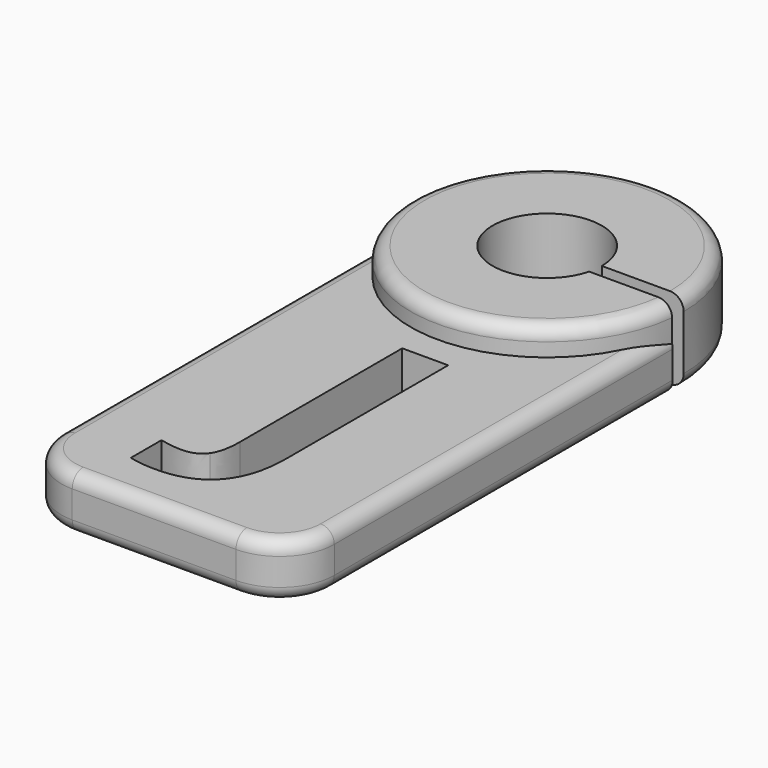
from build123d import *

# Parameters (mm, degrees)
F1_DEPTH     = 3
F2_DEPTH     = 2
F3_R         = 2
F4_T1_DEPTH  = 16.75
F4_T3_DEPTH  = 6
F4_T5_DEPTH  = 16
F4_T10_DEPTH = 16.75
F4_S11_R     = 5
F4_T12_DEPTH = 10
F4_T14_ANGLE = 359.64
F4_T18_DEPTH = 19.75
F4_S19_R     = 5
F4_T20_DEPTH = 11
F4_T22_ANGLE = 90
F4_T24_ANGLE = 90
F4_T26_ANGLE = 90
F4_T28_ANGLE = 180
F4_T30_ANGLE = 90


# Not quite as in the source:
# - a fillet or chamfer that OpenCascade refuses, or shapes differently, is made with other operations: its cross-section is extruded or revolved along the edge and cut away or added


with BuildPart() as f1:
    # F0 (on Top) → F1 (new body)
    with BuildSketch(Plane.XY):
        with BuildLine():
            Line((2, 0), (5, 0))
            ThreePointArc((5, 0), (0, 5), (-5, 0))
            ThreePointArc((-5, 0), (-0.2503138753, -4.9937303656), (4.9749371855, -0.5))
            Line((4.9749371855, -0.5), (1.9364916731, -0.5))
            ThreePointArc((1.9364916731, -0.5), (-1.9840593925, 0.252008585), (2, 0))
        make_face()
    extrude(amount=F1_DEPTH)

    # F0 (on Top) → F2 (join)
    with BuildSketch(Plane.XY):
        with BuildLine():
            ThreePointArc((4.9749371855, -0.5), (-0.2503138753, -4.9937303656), (-5, 0))
            Line((-5, 0), (-5, -18))
            Line((-5, -18), (5, -18))
            Line((5, -18), (5, -0.5))
            Line((5, -0.5), (4.9749371855, -0.5))
        make_face()
        with BuildLine():
            add(Edge.make_bspline(
                [(0.578588878, -15.5900442691), (-0.0559597331, -16.3174748247), (-1.2990152887, -16.3174748247)],
                knots=[0, 0, 0, 1, 1, 1], degree=2))
            add(Edge.make_bspline(
                [(-1.2990152887, -16.3174748247), (-1.8684597331, -16.3174748247), (-2.2920708442, -16.197683158)],
                knots=[0, 0, 0, 1, 1, 1], degree=2))
            Line((-2.2920708442, -16.197683158), (-2.2920708442, -14.7983776025))
            add(Edge.make_bspline(
                [(-2.2920708442, -14.7983776025), (-1.8580430665, -14.9060164914), (-1.5004041776, -14.9060164914)],
                knots=[0, 0, 0, 1, 1, 1], degree=2))
            add(Edge.make_bspline(
                [(-1.5004041776, -14.9060164914), (-0.9465847331, -14.9060164914), (-0.7078694553, -14.5613984358)],
                knots=[0, 0, 0, 1, 1, 1], degree=2))
            add(Edge.make_bspline(
                [(-0.7078694553, -14.5613984358), (-0.4691541776, -14.2167803802), (-0.4691541776, -13.4841414914)],
                knots=[0, 0, 0, 1, 1, 1], degree=2))
            Line((-0.4691541776, -13.4841414914), (-0.4691541776, -6.0518498247))
            Line((-0.4691541776, -6.0518498247), (1.2131374891, -6.0518498247))
            Line((1.2131374891, -6.0518498247), (1.2131374891, -13.4737248247))
            add(Edge.make_bspline(
                [(1.2131374891, -13.4737248247), (1.2131374891, -14.8626137136), (0.578588878, -15.5900442691)],
                knots=[0, 0, 0, 1, 1, 1], degree=2))
        make_face(mode=Mode.SUBTRACT)
    extrude(amount=F2_DEPTH)

    # F3
    f3_edges = [f1.edges().sort_by_distance(p)[0] for p in [
        (-5, -18, 1),
        (5, -18, 1),
    ]]
    fillet(f3_edges, radius=F3_R)

    # F4: fillet of radius 0.5 on 12 edges, made by hand

    # F4_s2 → F4_t1 (cut)
    with BuildSketch(Plane.XZ.offset(-0.75)):
        with BuildLine():
            ThreePointArc((5, 0.5), (4.8535533906, 0.1464466094), (4.5, 0))
            Line((4.5, 0), (5, 0))
            Line((5, 0), (5, 0.5))
        make_face()
    extrude(amount=F4_T1_DEPTH, mode=Mode.SUBTRACT)

    # F4_s4 → F4_t3 (cut)
    with BuildSketch(Plane.YZ.offset(-3)):
        with BuildLine():
            ThreePointArc((-17.5, 2), (-17.8535533906, 1.8535533906), (-18, 1.5))
            Line((-18, 1.5), (-18, 2))
            Line((-18, 2), (-17.5, 2))
        make_face()
        with BuildLine():
            ThreePointArc((-18, 0.5), (-17.8535533906, 0.1464466094), (-17.5, 0))
            Line((-17.5, 0), (-18, 0))
            Line((-18, 0), (-18, 0.5))
        make_face()
    extrude(amount=F4_T3_DEPTH, mode=Mode.SUBTRACT)

    # F4_s6 → F4_t5 (cut)
    with BuildSketch(Plane.XZ):
        with BuildLine():
            ThreePointArc((-5, 0.5), (-4.8535533906, 0.1464466094), (-4.5, 0))
            Line((-4.5, 0), (-5, 0))
            Line((-5, 0), (-5, 0.5))
        make_face()
    extrude(amount=F4_T5_DEPTH, mode=Mode.SUBTRACT)


with BuildPart() as f4_tool8:
    # F4_s9 → F4_t10 (new body)
    with BuildSketch(Plane.XZ.offset(16)):
        with BuildLine():
            ThreePointArc((4.5, 2), (4.8535533906, 1.8535533906), (5, 1.5))
            Line((5, 1.5), (5, 2))
            Line((5, 2), (4.5, 2))
        make_face()
    extrude(amount=-F4_T10_DEPTH)

    # F4_s11 → F4_t12 (cut, symmetric)
    with BuildSketch(Plane.XY.offset(1.8)):
        Circle(F4_S11_R)
    extrude(amount=F4_T12_DEPTH, both=True, mode=Mode.SUBTRACT)


with BuildPart() as f1_1:
    add(f1.part)

    # F4_t7: cut F4_tool8
    add(f4_tool8.part, mode=Mode.SUBTRACT)

    # F4_s13 → F4_t14 (revolve, cut)
    with BuildSketch(Plane(origin=(0, 0, 0), x_dir=(0, 0, 1), z_dir=(0.0532001762, 0.9985838679, 0))):
        with BuildLine():
            ThreePointArc((2.5, 5), (2.8535533906, 4.8535533906), (3, 4.5))
            Line((3, 4.5), (3, 5))
            Line((3, 5), (2.5, 5))
        make_face()
    revolve(axis=Axis((0, 0, 3), (0, 0, -1)), revolution_arc=F4_T14_ANGLE, mode=Mode.SUBTRACT)


with BuildPart() as f4_tool16:
    # F4_s17 → F4_t18 (new body)
    with BuildSketch(Plane.XZ.offset(-3.75)):
        with BuildLine():
            ThreePointArc((-4.5, 2), (-4.8535533906, 1.8535533906), (-5, 1.5))
            Line((-5, 1.5), (-5, 2))
            Line((-5, 2), (-4.5, 2))
        make_face()
    extrude(amount=F4_T18_DEPTH)

    # F4_s19 → F4_t20 (cut, symmetric)
    with BuildSketch(Plane.XY.offset(1.8)):
        Circle(F4_S19_R)
    extrude(amount=F4_T20_DEPTH, both=True, mode=Mode.SUBTRACT)


with BuildPart() as f1_2:
    add(f1_1.part)

    # F4_t15: cut F4_tool16
    add(f4_tool16.part, mode=Mode.SUBTRACT)

    # F4_s21 → F4_t22 (revolve, cut)
    with BuildSketch(Plane.YZ.offset(-3)):
        with BuildLine():
            ThreePointArc((-17.5, 2), (-17.8535533906, 1.8535533906), (-18, 1.5))
            Line((-18, 1.5), (-18, 2))
            Line((-18, 2), (-17.5, 2))
        make_face()
    revolve(axis=Axis((-3, -16, 2), (0, 0, -1)), revolution_arc=F4_T22_ANGLE, mode=Mode.SUBTRACT)

    # F4_s23 → F4_t24 (revolve, cut)
    with BuildSketch(Plane.YZ.offset(3)):
        with BuildLine():
            ThreePointArc((-17.5, 2), (-17.8535533906, 1.8535533906), (-18, 1.5))
            Line((-18, 1.5), (-18, 2))
            Line((-18, 2), (-17.5, 2))
        make_face()
    revolve(axis=Axis((3, -16, 2), (0, 0, 1)), revolution_arc=F4_T24_ANGLE, mode=Mode.SUBTRACT)

    # F4_s25 → F4_t26 (revolve, cut)
    with BuildSketch(Plane.YZ.offset(-3)):
        with BuildLine():
            ThreePointArc((-18, 0.5), (-17.8535533906, 0.1464466094), (-17.5, 0))
            Line((-17.5, 0), (-18, 0))
            Line((-18, 0), (-18, 0.5))
        make_face()
    revolve(axis=Axis((-3, -16, 0), (0, 0, -1)), revolution_arc=F4_T26_ANGLE, mode=Mode.SUBTRACT)

    # F4_s27 → F4_t28 (revolve, cut)
    with BuildSketch(Plane.XZ):
        with BuildLine():
            ThreePointArc((5, 0.5), (4.8535533906, 0.1464466094), (4.5, 0))
            Line((4.5, 0), (5, 0))
            Line((5, 0), (5, 0.5))
        make_face()
    revolve(axis=Axis((0, 0, 0), (0, 0, 1)), revolution_arc=F4_T28_ANGLE, mode=Mode.SUBTRACT)

    # F4_s29 → F4_t30 (revolve, cut)
    with BuildSketch(Plane.YZ.offset(3)):
        with BuildLine():
            ThreePointArc((-18, 0.5), (-17.8535533906, 0.1464466094), (-17.5, 0))
            Line((-17.5, 0), (-18, 0))
            Line((-18, 0), (-18, 0.5))
        make_face()
    revolve(axis=Axis((3, -16, 0), (0, 0, 1)), revolution_arc=F4_T30_ANGLE, mode=Mode.SUBTRACT)


solid = f1_2.part
